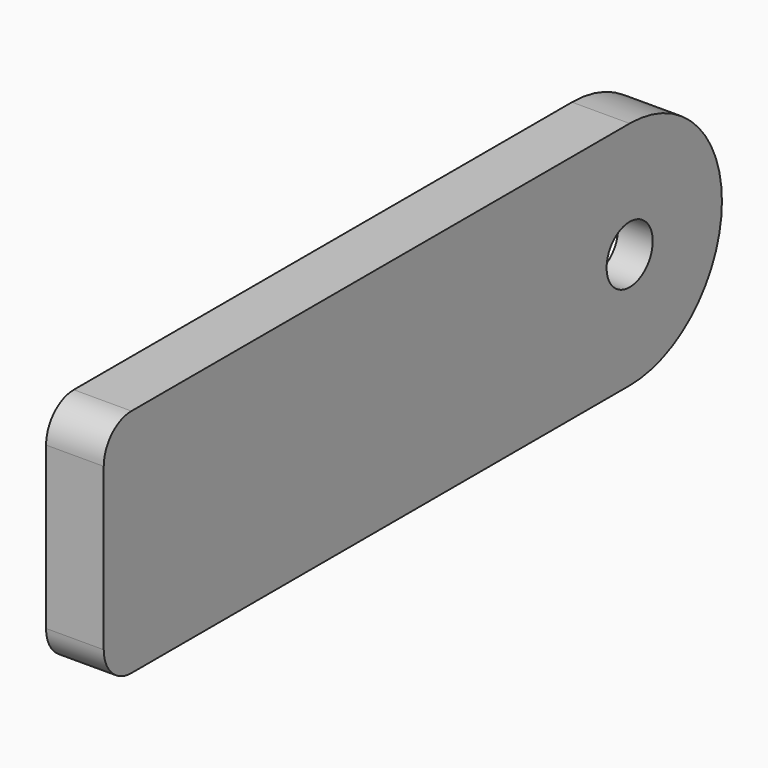
from build123d import *

# Parameters (mm, degrees)
F0_R         = 2.5
F1_DEPTH     = 3
F2_TEXT_SIZE = 12.5
F3_DEPTH     = 1
F5_DEPTH     = 2


# Not quite as in the source:
# - Text() gives the source's letters only with a copy of the font that has no kerning and outlines rounded to 1/6400 em; it was checked with that copy


with BuildPart() as f1:
    # F0 (on Right) → F1 (new body)
    with BuildSketch(Plane.YZ):
        with BuildLine():
            ThreePointArc((-33.5, -7), (-32.6213203436, -9.1213203436), (-30.5, -10))
            Line((-30.5, -10), (23.5, -10))
            ThreePointArc((23.5, -10), (33.5, 0), (23.5, 10))
            Line((23.5, 10), (-30.5, 10))
            ThreePointArc((-30.5, 10), (-32.6213203436, 9.1213203436), (-33.5, 7))
            Line((-33.5, 7), (-33.5, -7))
        make_face()
        with Locations((23.5, 0)):
            Circle(F0_R, mode=Mode.SUBTRACT)
    extrude(amount=F1_DEPTH)

    # F2 (on face) → F3 (join)
    with BuildSketch(Plane(origin=(0, 0, 0), x_dir=(0, -1, 0), z_dir=(-1, 0, 0))):
        with Locations((-16.390625, -4.5)):
            Text('semere', F2_TEXT_SIZE, font='Open Sans', text_align=(TextAlign.LEFT, TextAlign.BOTTOM))
    extrude(amount=F3_DEPTH)

    # F4 (on face) → F5 (join)
    with BuildSketch(Plane(origin=(0, 0, 0), x_dir=(0, -1, 0), z_dir=(-1, 0, 0))):
        with BuildLine():
            Line((-23.5, -10), (30.5, -10))
            ThreePointArc((30.5, -10), (32.6213203436, -9.1213203436), (33.5, -7))
            Line((33.5, -7), (33.5, 7))
            ThreePointArc((33.5, 7), (32.6213203436, 9.1213203436), (30.5, 10))
            Line((30.5, 10), (-23.5, 10))
            ThreePointArc((-23.5, 10), (-33.5, 0), (-23.5, -10))
        make_face()
        with BuildLine():
            ThreePointArc((30.5, 8.5481852293), (31.5947322742, 8.0947322742), (32.0481852293, 7))
            Line((32.0481852293, 7), (32.0481852293, -7))
            ThreePointArc((32.0481852293, -7), (31.5947322742, -8.0947322742), (30.5, -8.5481852293))
            Line((30.5, -8.5481852293), (-23.5, -8.5481852293))
            ThreePointArc((-23.5, -8.5481852293), (-32.0481852293, 0), (-23.5, 8.5481852293))
            Line((-23.5, 8.5481852293), (30.5, 8.5481852293))
        make_face(mode=Mode.SUBTRACT)
    extrude(amount=F5_DEPTH)


solid = f1.part
